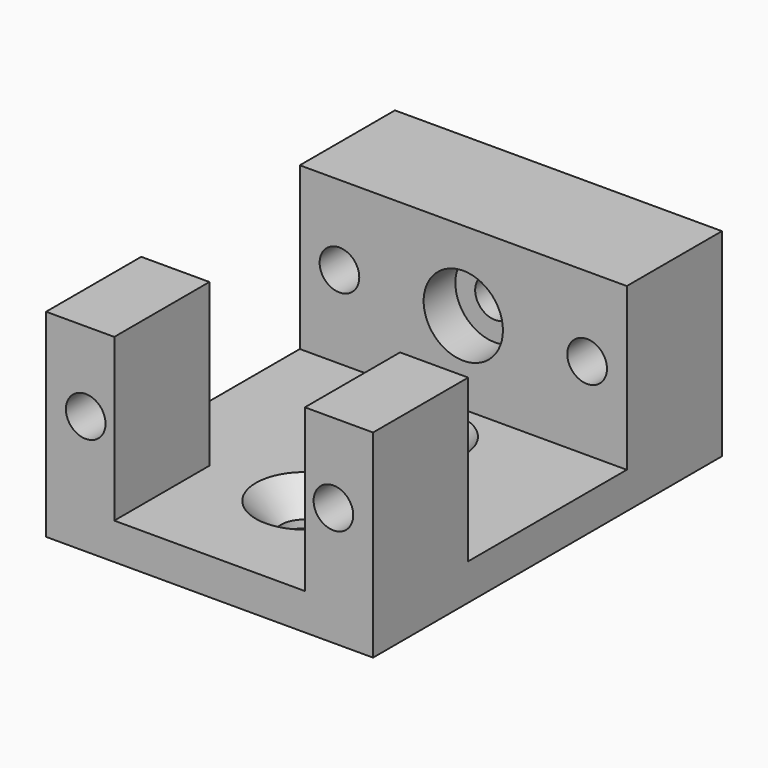
from build123d import *

# Parameters (mm, degrees)
F0_W           = 26.1874
F0_H           = 34.925
F1_DEPTH       = 15.875
F3_DEPTH       = 12.954
F4_R           = 1.5875
F5_DEPTH       = 34.926
F6_R           = 1.5875
F7_DEPTH       = 9.526
F9_D           = 3.7973
F9_CSINK_D     = 7.7978
F9_CSINK_ANGLE = 82
F10_R          = 3.175
F10_R_2        = 1.5875
F11_DEPTH      = 3.175


with BuildPart() as f1:
    # F0 (on Top) → F1 (new body)
    with BuildSketch(Plane.XY):
        with Locations((13.0937, 17.4625)):
            Rectangle(F0_W, F0_H)
    extrude(amount=F1_DEPTH)

    # F2 (on face) → F3 (cut)
    with BuildSketch(Plane.XY.offset(15.875)):
        Polygon((26.1874, 25.4), (0, 25.4), (0, 9.525), (5.461, 9.525), (5.461, 0), (20.7264, 0), (20.7264, 9.525), (26.1874, 9.525), align=None)
    extrude(amount=-F3_DEPTH, mode=Mode.SUBTRACT)

    # F4 (on face) → F5 (cut, through all)
    with BuildSketch(Plane.XZ):
        with Locations((3.175, 9.525)):
            Circle(F4_R)
        with Locations((23.0124, 9.525)):
            Circle(F4_R)
    extrude(amount=-F5_DEPTH, mode=Mode.SUBTRACT)

    # F6 (on face) → F7 (cut, through all)
    with BuildSketch(Plane.XZ.offset(-25.4)):
        with Locations((13.0937, 9.525)):
            Circle(F6_R)
    extrude(amount=-F7_DEPTH, mode=Mode.SUBTRACT)

    # F9 (through all)
    with Locations(Plane.XY.offset(2.921)):
        with Locations((13.081, 20.6502), (13.081, 9.525)):
            CounterSinkHole(F9_D / 2, F9_CSINK_D / 2, counter_sink_angle=F9_CSINK_ANGLE)

    # F10 (on face) → F11 (cut)
    with BuildSketch(Plane.XZ.offset(-25.4)):
        with Locations((13.0937, 9.525)):
            Circle(F10_R)
        with Locations((13.0937, 9.525)):
            Circle(F10_R_2, mode=Mode.SUBTRACT)
    extrude(amount=-F11_DEPTH, mode=Mode.SUBTRACT)


solid = f1.part
